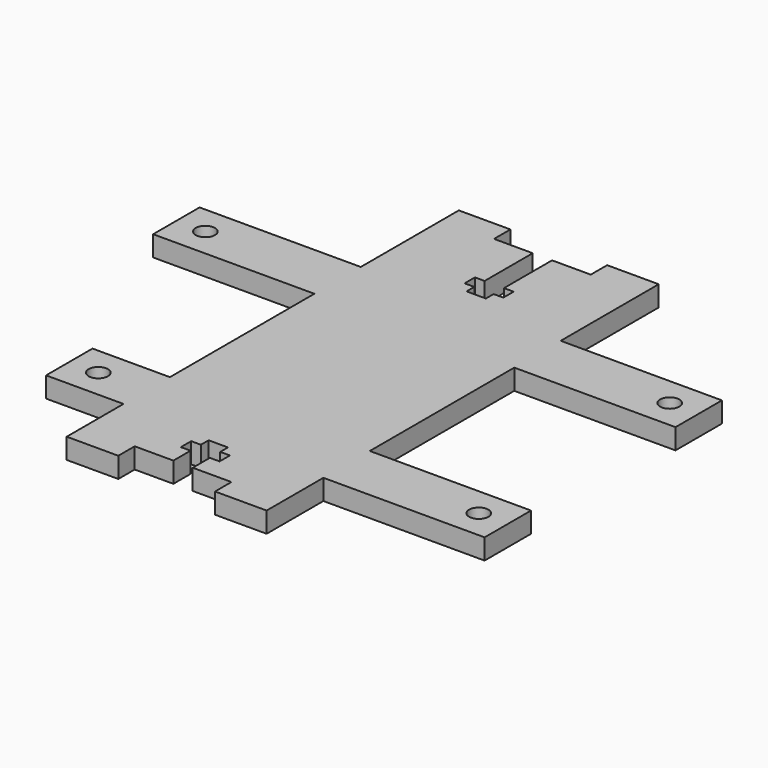
from build123d import *

# Parameters (mm, degrees)
F0_R     = 1.5
F0_W     = 8
F0_H     = 3.175
F0_W_2   = 31
F0_H_2   = 9
F0_W_3   = 12
F0_W_4   = 25
F1_DEPTH = 3.175


# Not quite as in the source:
# - a length typed as a fraction of an inch, garbled in the dataset ("3 / 203.2 mm" for 3/8 in), is restored
# - a feature names something its author has since deleted; it is built from what else it names


with BuildPart() as f1:
    # F0 (on Top) → F1 (new body)
    with BuildSketch(Plane.XY):
        Polygon((7.0042573512, 24.8119444549), (-17.9957426488, 24.8119444549), (-17.9957426488, 15.8119444549), (7.0042573512, 15.8119444549), (22.5042573512, 15.8119444549), (38.0042573512, 15.8119444549), (63.0042573512, 15.8119444549), (63.0042573512, 24.8119444549), (38.0042573512, 24.8119444549), align=None)
        with Locations((-13.4957426488, 20.3119444549)):
            Circle(F0_R, mode=Mode.SUBTRACT)
        with Locations((58.5042573512, 20.3119444549)):
            Circle(F0_R, mode=Mode.SUBTRACT)
        Polygon((7.0042573512, 40.6369444549), (7.0042573512, 24.8119444549), (38.0042573512, 24.8119444549), (38.0042573512, 40.6369444549), (30.0042573512, 40.6369444549), (24.0042573512, 40.6369444549), (24.0042573512, 31.3119444549), (25.5042573512, 31.3119444549), (25.5042573512, 29.3119444549), (24.0042573512, 29.3119444549), (24.0042573512, 27.8119444549), (21.0042573512, 27.8119444549), (21.0042573512, 29.3119444549), (19.5042573512, 29.3119444549), (19.5042573512, 31.3119444549), (21.0042573512, 31.3119444549), (21.0042573512, 40.6369444549), (15.0042573512, 40.6369444549), align=None)
        with Locations((11.0042573512, 42.2244444549)):
            Rectangle(F0_W, F0_H)
        Polygon((22.5042573512, 15.8119444549), (7.0042573512, 15.8119444549), (7.0042573512, -12.1880555451), (38.0042573512, -12.1880555451), (38.0042573512, 15.8119444549), align=None)
        with Locations((34.0042573512, 42.2244444549)):
            Rectangle(F0_W, F0_H)
        with Locations((22.5042573512, -16.6880555451)):
            Rectangle(F0_W_2, F0_H_2)
        with Locations((1.0042573512, -16.6880555451)):
            Rectangle(F0_W_3, F0_H_2)
        with Locations((-0.4957426488, -16.6880555451)):
            Circle(F0_R, mode=Mode.SUBTRACT)
        Polygon((38.0042573512, -21.1880555451), (7.0042573512, -21.1880555451), (7.0042573512, -29.0130555451), (15.0042573512, -29.0130555451), (21.0042573512, -29.0130555451), (21.0042573512, -25.6880555451), (19.5042573512, -25.6880555451), (19.5042573512, -23.6880555451), (21.0042573512, -23.6880555451), (21.0042573512, -22.1880555451), (24.0042573512, -22.1880555451), (24.0042573512, -23.6880555451), (25.5042573512, -23.6880555451), (25.5042573512, -25.6880555451), (24.0042573512, -25.6880555451), (24.0042573512, -29.0130555451), (30.0042573512, -29.0130555451), (38.0042573512, -29.0130555451), align=None)
        with Locations((50.5042573512, -16.6880555451)):
            Rectangle(F0_W_4, F0_H_2)
        with Locations((58.5042573512, -16.6880555451)):
            Circle(F0_R, mode=Mode.SUBTRACT)
        with Locations((11.0042573512, -30.6005555451)):
            Rectangle(F0_W, F0_H)
        with Locations((34.0042573512, -30.6005555451)):
            Rectangle(F0_W, F0_H)
    extrude(amount=F1_DEPTH)


solid = f1.part
